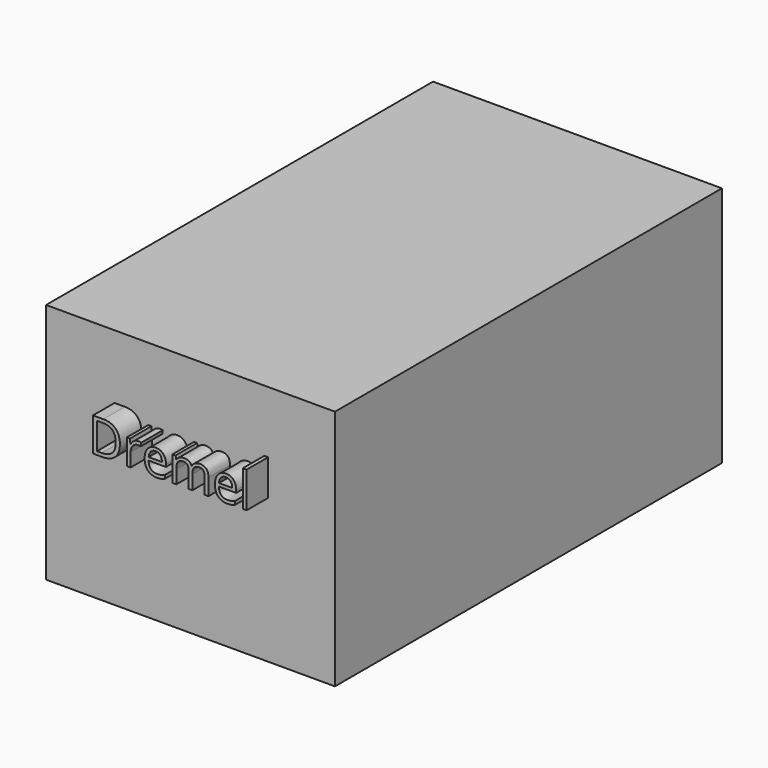
from build123d import *

# Parameters (mm, degrees)
F0_W         = 273.05
F0_H         = 228.6
F1_DEPTH     = 457.2
F2_TEXT_SIZE = 44.5410539775
F3_DEPTH     = 25.4


# Not quite as in the source:
# - Text() gives the source's letters only with a copy of the font that has no kerning and outlines rounded to 1/6400 em; it was checked with that copy


with BuildPart() as f1:
    # F0 (on Front) → F1 (new body)
    with BuildSketch(Plane.XZ):
        Rectangle(F0_W, F0_H)
    extrude(amount=F1_DEPTH)

    # F2 (on face) → F3 (join)
    with BuildSketch(Plane.XZ.offset(457.2)):
        with Locations((-76.2, 21.9868134954)):
            Text('Dremel', F2_TEXT_SIZE, font='Open Sans', text_align=(TextAlign.LEFT, TextAlign.BOTTOM))
    extrude(amount=F3_DEPTH)


solid = f1.part
